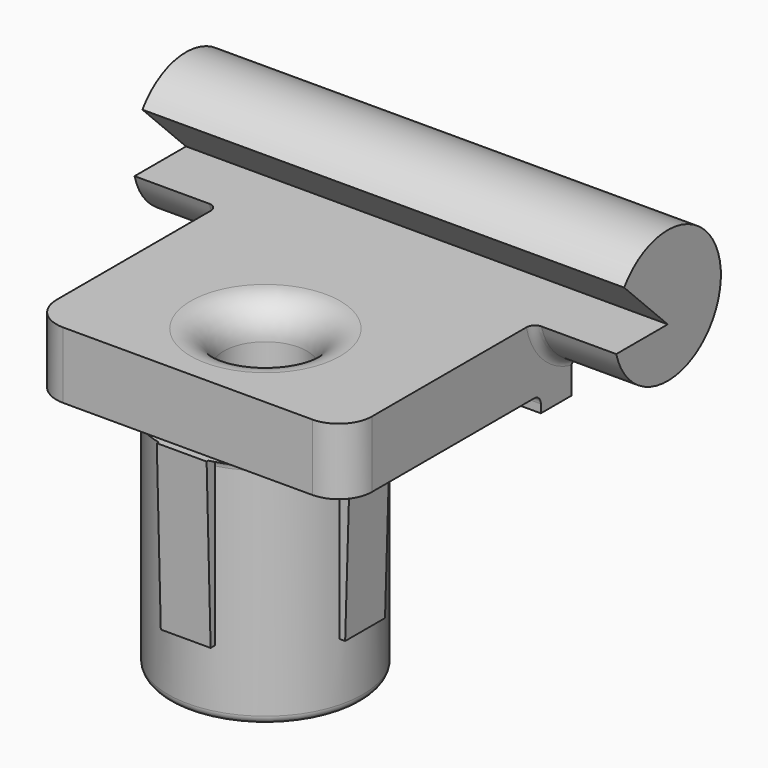
from build123d import *

# Parameters (mm, degrees)
F0_R            = 5.85
F1_DEPTH        = 14
F2_W            = 19
F2_H            = 17
F3_DEPTH        = 4
F4_W            = 19
F4_H            = 2.3
F5_DEPTH        = 1
F7_DEPTH        = 1.5
F7_COPIES_COUNT = 4
F9_DEPTH        = 14.5
F10_R           = 2.5
F11_DEPTH       = 15
F12_R           = 2
F13_T1_DEPTH    = 19
F13_T6_ANGLE    = 84.7754573572
F13_T12_ANGLE   = 84.7754573572
F13_T18_ANGLE   = 84.7754573572
F13_T24_ANGLE   = 84.7754573572
F13_T30_ANGLE   = 96.86145484
F13_T36_ANGLE   = 96.86145484
F13_T43_ANGLE   = 96.86145484
F13_T47_DEPTH   = 20.497881522
F13_T54_ANGLE   = 96.86145484
F13_T58_DEPTH   = 20.497881522


# Not quite as in the source:
# - a fillet or chamfer that OpenCascade refuses, or shapes differently, is made with other operations: its cross-section is extruded or revolved along the edge and cut away or added
# - a pattern or mirror of a feature is missing from the dataset's text; its kind, count and spacing are read off the source's solid


with BuildPart() as f1:
    # F0 (on Top) → F1 (new body)
    with BuildSketch(Plane.XY):
        Circle(F0_R)
    extrude(amount=-F1_DEPTH)

    # F2 (on Top) → F3 (join)
    with BuildSketch(Plane.XY):
        with Locations((0, 2.65)):
            Rectangle(F2_W, F2_H)
    extrude(amount=F3_DEPTH)

    # F4 (on Top) → F5 (join)
    with BuildSketch(Plane.XY):
        with Locations((0, 10)):
            Rectangle(F4_W, F4_H)
    extrude(amount=-F5_DEPTH)

    # F6 (on Front) → F7 (join, symmetric)
    with BuildSketch(Plane.XZ):
        Polygon((6, -10), (6.3, 0), (5, 0), (5, -10), align=None)
    f7 = extrude(amount=F7_DEPTH, both=True)

    # F7_copies: F7 ×4 about axis
    f7_copies_axis = Axis((0, 0, 0), (0, 0, 1))
    for i in range(1, F7_COPIES_COUNT):
        add(f7.rotate(f7_copies_axis, i * 360 / F7_COPIES_COUNT))

    # F8 (on Right) → F9 (join, symmetric)
    with BuildSketch(Plane.YZ):
        with BuildLine():
            Line((12.15, 4), (8.2770166538, 4))
            ThreePointArc((8.2770166538, 4), (16.0871501864, 4.2937079857), (8.8661178186, 7.2838821814))
            Line((8.8661178186, 7.2838821814), (12.15, 4))
        make_face()
    extrude(amount=F9_DEPTH, both=True)

    # F10 (on Top) → F11 (cut, symmetric)
    with BuildSketch(Plane.XY):
        Circle(F10_R)
    extrude(amount=F11_DEPTH, both=True, mode=Mode.SUBTRACT)

    # F12
    f12_edges = [f1.edges().sort_by_distance(p)[0] for p in [
        (-9.5, -5.85, 2),
        (9.5, -5.85, 2),
        (-2.5, 0, -14),
        (-2.5, 0, 4),
    ]]
    fillet(f12_edges, radius=F12_R)

    # F13: fillet of radius 0.5 on 9 edges, made by hand

    # F13_s2 → F13_t1 (join)
    with BuildSketch(Plane.YZ.offset(-9.5)):
        with BuildLine():
            ThreePointArc((8.35, 0), (8.7035533906, -0.1464466094), (8.85, -0.5))
            Line((8.85, -0.5), (8.85, 0))
            Line((8.85, 0), (8.35, 0))
        make_face()
        with BuildLine():
            ThreePointArc((11.7055555556, 1.02476804), (11.3166666667, 0.9005420413), (11.15, 0.527864045))
            Line((11.15, 0.527864045), (11.15, 1.1270166538))
            ThreePointArc((11.15, 1.1270166538), (11.4259705579, 1.0660730349), (11.7055555556, 1.02476804))
        make_face()
    extrude(amount=F13_T1_DEPTH)


with BuildPart() as f13_tool4:
    # F13_s5 → F13_t6 (revolve)
    with BuildSketch(Plane(origin=(0, 0, 0), x_dir=(0, 0, 1), z_dir=(-0.9989608313, -0.0455769416, 0))):
        with BuildLine():
            ThreePointArc((0, -6.35), (-0.1464466094, -5.9964466094), (-0.5, -5.85))
            Line((-0.5, -5.85), (0, -5.85))
            Line((0, -5.85), (0, -6.35))
        make_face()
    revolve(axis=Axis((0, 0, 0), (0, 0, 1)), revolution_arc=F13_T6_ANGLE)

    split(bisect_by=Plane(origin=(6.2943350984, 0, -0.188830053), x_dir=(0, 1, 0), z_dir=(-0.9995503035, 0, 0.0299865091)), keep=Keep.TOP)

    split(bisect_by=Plane(origin=(0, -6.2943350984, -0.188830053), x_dir=(1, 0, 0), z_dir=(0, 0.9995503035, 0.0299865091)), keep=Keep.TOP)


with BuildPart() as f1_1:
    add(f1.part)

    # F13_t3: union F13_tool4
    add(f13_tool4.part)


with BuildPart() as f13_tool10:
    # F13_s11 → F13_t12 (revolve)
    with BuildSketch(Plane(origin=(0, 0, 0), x_dir=(0, 0, 1), z_dir=(0.0455769416, -0.9989608313, 0))):
        with BuildLine():
            ThreePointArc((0, -6.35), (-0.1464466094, -5.9964466094), (-0.5, -5.85))
            Line((-0.5, -5.85), (0, -5.85))
            Line((0, -5.85), (0, -6.35))
        make_face()
    revolve(axis=Axis((0, 0, 0), (0, 0, 1)), revolution_arc=F13_T12_ANGLE)

    split(bisect_by=Plane.XZ.offset(-1.5), keep=Keep.BOTTOM)

    split(bisect_by=Plane(origin=(0, 6.2943350984, -0.188830053), x_dir=(1, 0, 0), z_dir=(0, -0.9995503035, 0.0299865091)), keep=Keep.TOP)


with BuildPart() as f1_2:
    add(f1_1.part)

    # F13_t9: union F13_tool10
    add(f13_tool10.part)


with BuildPart() as f13_tool16:
    # F13_s17 → F13_t18 (revolve)
    with BuildSketch(Plane(origin=(0, 0, 0), x_dir=(0, 0, 1), z_dir=(0.9989608313, 0.0455769416, 0))):
        with BuildLine():
            ThreePointArc((0, -6.35), (-0.1464466094, -5.9964466094), (-0.5, -5.85))
            Line((-0.5, -5.85), (0, -5.85))
            Line((0, -5.85), (0, -6.35))
        make_face()
    revolve(axis=Axis((0, 0, 0), (0, 0, 1)), revolution_arc=F13_T18_ANGLE)

    split(bisect_by=Plane.XZ.offset(-1.5), keep=Keep.BOTTOM)

    split(bisect_by=Plane.YZ.offset(-1.5), keep=Keep.BOTTOM)


with BuildPart() as f1_3:
    add(f1_2.part)

    # F13_t15: union F13_tool16
    add(f13_tool16.part)


with BuildPart() as f13_tool22:
    # F13_s23 → F13_t24 (revolve)
    with BuildSketch(Plane(origin=(0, 0, 0), x_dir=(0, 0, 1), z_dir=(-0.0455769416, 0.9989608313, 0))):
        with BuildLine():
            ThreePointArc((0, -6.35), (-0.1464466094, -5.9964466094), (-0.5, -5.85))
            Line((-0.5, -5.85), (0, -5.85))
            Line((0, -5.85), (0, -6.35))
        make_face()
    revolve(axis=Axis((0, 0, 0), (0, 0, 1)), revolution_arc=F13_T24_ANGLE)

    split(bisect_by=Plane(origin=(-6.2943350984, 0, -0.188830053), x_dir=(0, 1, 0), z_dir=(0.9995503035, 0, 0.0299865091)), keep=Keep.TOP)

    split(bisect_by=Plane(origin=(0, -6.2943350984, -0.188830053), x_dir=(1, 0, 0), z_dir=(0, 0.9995503035, 0.0299865091)), keep=Keep.TOP)


with BuildPart() as f1_4:
    add(f1_3.part)

    # F13_t21: union F13_tool22
    add(f13_tool22.part)


with BuildPart() as f13_tool28:
    # F13_s29 → F13_t30 (revolve)
    with BuildSketch(Plane(origin=(0, 0.3421818863, 5.7078686812), x_dir=(1, 0, 0), z_dir=(0, 0.0598417157, 0.9982078787))):
        with BuildLine():
            ThreePointArc((-9.5, 7.3290171475), (-9.6464466094, 7.6825705381), (-10, 7.8290171475))
            Line((-10, 7.8290171475), (-9.5, 7.8290171475))
            Line((-9.5, 7.8290171475), (-9.5, 7.3290171475))
        make_face()
    revolve(axis=Axis((-9.5, 12.15, 5), (1, 0, 0)), revolution_arc=F13_T30_ANGLE)

    split(bisect_by=Plane.XY.offset(4), keep=Keep.BOTTOM)

    split(bisect_by=Plane.XZ.offset(-11.15), keep=Keep.TOP)


with BuildPart() as f1_5:
    add(f1_4.part)

    # F13_t27: union F13_tool28
    add(f13_tool28.part)


with BuildPart() as f13_tool34:
    # F13_s35 → F13_t36 (revolve)
    with BuildSketch(Plane(origin=(0, 0.3421818863, 5.7078686812), x_dir=(1, 0, 0), z_dir=(0, 0.0598417157, 0.9982078787))):
        with BuildLine():
            ThreePointArc((9.5, 7.3290171475), (9.6464466094, 7.6825705381), (10, 7.8290171475))
            Line((10, 7.8290171475), (9.5, 7.8290171475))
            Line((9.5, 7.8290171475), (9.5, 7.3290171475))
        make_face()
    revolve(axis=Axis((9.5, 12.15, 5), (1, 0, 0)), revolution_arc=F13_T36_ANGLE)

    split(bisect_by=Plane.XY.offset(4), keep=Keep.BOTTOM)

    split(bisect_by=Plane.XZ.offset(-11.15), keep=Keep.TOP)


with BuildPart() as f1_6:
    add(f1_5.part)

    # F13_t33: union F13_tool34
    add(f13_tool34.part)


with BuildPart() as f13_tool41:
    # F13_s42 → F13_t43 (revolve)
    with BuildSketch(Plane(origin=(0, 0.3421818863, 5.7078686812), x_dir=(1, 0, 0), z_dir=(0, 0.0598417157, 0.9982078787))):
        with BuildLine():
            ThreePointArc((-9.5, 7.3290171475), (-9.6464466094, 7.6825705381), (-10, 7.8290171475))
            Line((-10, 7.8290171475), (-9.5, 7.8290171475))
            Line((-9.5, 7.8290171475), (-9.5, 7.3290171475))
        make_face()
    revolve(axis=Axis((-9.5, 12.15, 5), (1, 0, 0)), revolution_arc=F13_T43_ANGLE)

    split(bisect_by=Plane.XZ.offset(-11.15), keep=Keep.BOTTOM)


with BuildPart() as f13_tool45:
    # F13_s46 → F13_t47 (new body)
    with BuildSketch(Plane.YZ.offset(-10.997881522)):
        with BuildLine():
            ThreePointArc((11.7055555556, 1.02476804), (11.3166666667, 0.9005420413), (11.15, 0.527864045))
            Line((11.15, 0.527864045), (11.15, 1.1270166538))
            ThreePointArc((11.15, 1.1270166538), (11.4259705579, 1.0660730349), (11.7055555556, 1.02476804))
        make_face()
    extrude(amount=F13_T47_DEPTH)

    split(bisect_by=Plane.YZ.offset(-9.5), keep=Keep.BOTTOM)


with BuildPart() as f13_tool41_1:
    add(f13_tool41.part)

    # F13_t49: intersect F13_tool45
    add(f13_tool45.part, mode=Mode.INTERSECT)


with BuildPart() as f1_7:
    add(f1_6.part)

    # F13_t39: union F13_tool41
    add(f13_tool41_1.part)


with BuildPart() as f13_tool52:
    # F13_s53 → F13_t54 (revolve)
    with BuildSketch(Plane(origin=(0, 0.3421818863, 5.7078686812), x_dir=(1, 0, 0), z_dir=(0, 0.0598417157, 0.9982078787))):
        with BuildLine():
            ThreePointArc((9.5, 7.3290171475), (9.6464466094, 7.6825705381), (10, 7.8290171475))
            Line((10, 7.8290171475), (9.5, 7.8290171475))
            Line((9.5, 7.8290171475), (9.5, 7.3290171475))
        make_face()
    revolve(axis=Axis((9.5, 12.15, 5), (1, 0, 0)), revolution_arc=F13_T54_ANGLE)

    split(bisect_by=Plane.XZ.offset(-11.15), keep=Keep.BOTTOM)


with BuildPart() as f13_tool56:
    # F13_s57 → F13_t58 (new body)
    with BuildSketch(Plane.YZ.offset(-9.5)):
        with BuildLine():
            ThreePointArc((11.7055555556, 1.02476804), (11.3166666667, 0.9005420413), (11.15, 0.527864045))
            Line((11.15, 0.527864045), (11.15, 1.1270166538))
            ThreePointArc((11.15, 1.1270166538), (11.4259705579, 1.0660730349), (11.7055555556, 1.02476804))
        make_face()
    extrude(amount=F13_T58_DEPTH)

    split(bisect_by=Plane.YZ.offset(9.5), keep=Keep.TOP)


with BuildPart() as f13_tool52_1:
    add(f13_tool52.part)

    # F13_t60: intersect F13_tool56
    add(f13_tool56.part, mode=Mode.INTERSECT)


with BuildPart() as f1_8:
    add(f1_7.part)

    # F13_t50: union F13_tool52
    add(f13_tool52_1.part)

    # F13_s61 → F13_t62 (revolve, cut)
    with BuildSketch(Plane.XZ):
        with BuildLine():
            ThreePointArc((5.85, -13.5), (5.7035533906, -13.8535533906), (5.35, -14))
            Line((5.35, -14), (5.85, -14))
            Line((5.85, -14), (5.85, -13.5))
        make_face()
    revolve(axis=Axis((0, 0, -14), (0, 0, 1)), mode=Mode.SUBTRACT)


solid = f1_8.part
